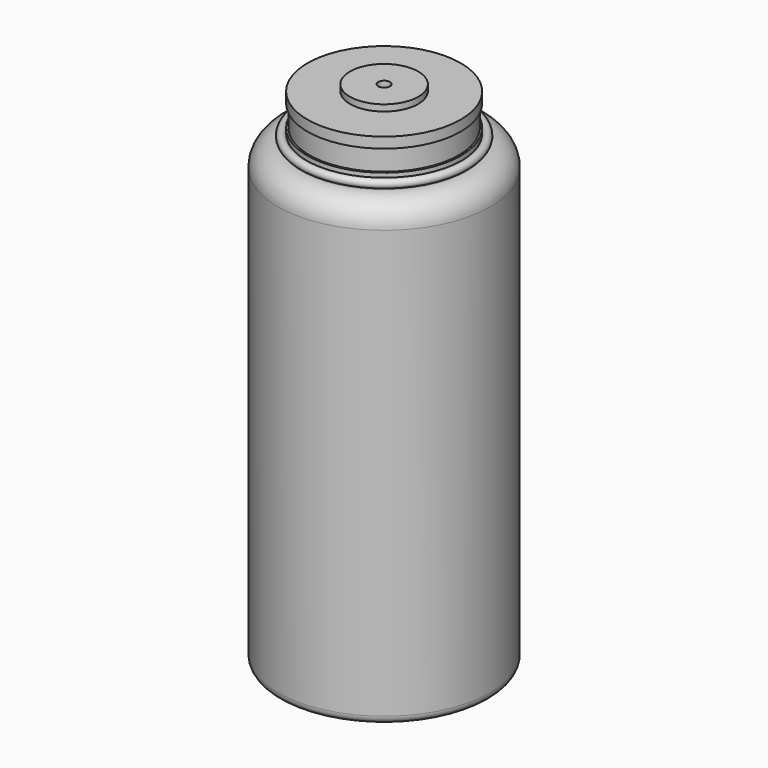
from build123d import *

# Parameters (mm, degrees)
F0_W      = 45
F0_H      = 195
F2_R      = 10
F3_R      = 35
F4_DEPTH  = 5
F5_R      = 7.1585667821
F6_DEPTH  = 5
F5_R_2    = 15.6792313498
F7_DEPTH  = 2.5
F8_R      = 1.8
F11_R     = 32.5
F12_DEPTH = 5
F13_R     = 31.75
F14_DEPTH = 9
F15_R     = 32.5
F16_DEPTH = 4.5
F17_R     = 14.5
F18_DEPTH = 2.7
F19_R     = 2.5
F20_DEPTH = 2.5
F21_R     = 3.5


# Not quite as in the source:
# - the program builds the solid bodies; features that only make, move or delete a surface that nothing else refers to are left out


with BuildPart() as f1:
    # F0 (on Front) → F1 (revolve)
    with BuildSketch(Plane.XZ):
        with Locations((38.1859867275, 23.317027688)):
            Rectangle(F0_W, F0_H)
    revolve(axis=Axis((15.6859867275, 0, 23.317027688), (0, 0, -1)))

    # F2
    f2_edges = [f1.edges().sort_by_distance(p)[0] for p in [
        (-29.314013, 0, 120.817028),
    ]]
    fillet(f2_edges, radius=F2_R)

    # F3 (on face) → F4 (cut)
    with BuildSketch(Plane(origin=(0, 0, -74.182972312), x_dir=(1, 0, 0), z_dir=(0, 0, -1))):
        with Locations((15.6859867275, 0)):
            Circle(F3_R)
    extrude(amount=-F4_DEPTH, mode=Mode.SUBTRACT)

    # F5 (on face) → F6 (cut)
    with BuildSketch(Plane(origin=(0, 0, -69.182972312), x_dir=(1, 0, 0), z_dir=(0, 0, -1))):
        with Locations((15.6859867275, 0)):
            Circle(F5_R)
    extrude(amount=-F6_DEPTH, mode=Mode.SUBTRACT)

    # F5 (on face) → F7 (cut)
    with BuildSketch(Plane(origin=(0, 0, -69.182972312), x_dir=(1, 0, 0), z_dir=(0, 0, -1))):
        with Locations((15.6859867275, 0)):
            Circle(F5_R_2)
        with Locations((15.6859867275, 0)):
            Circle(F5_R, mode=Mode.SUBTRACT)
    extrude(amount=-F7_DEPTH, mode=Mode.SUBTRACT)

    # F21
    f21_edges = [f1.edges().sort_by_distance(p)[0] for p in [
        (-29.314013, 0, -74.182972),
    ]]
    fillet(f21_edges, radius=F21_R)


with BuildPart() as f10:
    # F10: sweep along a path in F9
    with BuildLine(Plane.XY.offset(120.817027688)) as f10_path:
        CenterArc((15.6859867275, 0), 35, 0, 360)
    # F8 (on Front) → F10 (sweep)
    with BuildSketch(Plane.XZ):
        with Locations((49.783539027, 122.7821856737)):
            Circle(F8_R)
    sweep(path=f10_path.line)


with BuildPart() as f12:
    # F11 (on face) → F12 (new body)
    with BuildSketch(Plane.XY.offset(120.817027688)):
        with Locations((15.6859867275, 0)):
            Circle(F11_R)
    extrude(amount=F12_DEPTH)

    # F13 (on face) → F14 (join)
    with BuildSketch(Plane.XY.offset(125.817027688)):
        with Locations((15.6859867275, 0)):
            Circle(F13_R)
    extrude(amount=F14_DEPTH)


with BuildPart() as f16:
    # F15 (on face) → F16 (new body)
    with BuildSketch(Plane.XY.offset(134.817027688)):
        with Locations((15.6859867275, 0)):
            Circle(F15_R)
    extrude(amount=F16_DEPTH)


with BuildPart() as f18:
    # F17 (on face) → F18 (new body)
    with BuildSketch(Plane.XY.offset(139.317027688)):
        with Locations((15.6859867275, 0)):
            Circle(F17_R)
    extrude(amount=F18_DEPTH)

    # F19 (on face) → F20 (cut)
    with BuildSketch(Plane.XY.offset(142.017027688)):
        with Locations((15.6859867275, 0)):
            Circle(F19_R)
    extrude(amount=-F20_DEPTH, mode=Mode.SUBTRACT)


solid = Compound([f1.part, f10.part, f12.part, f16.part, f18.part])
